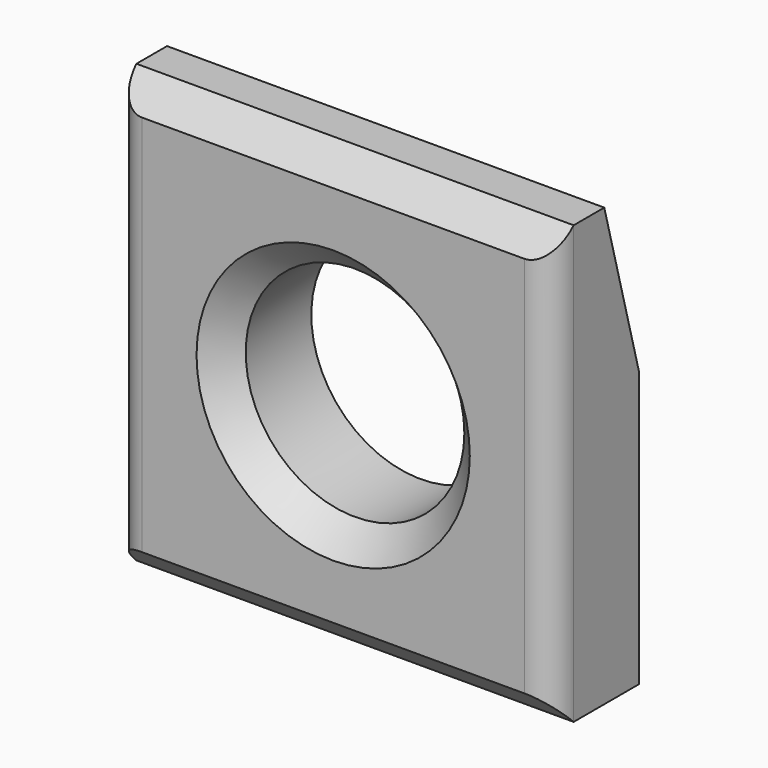
from build123d import *

# Parameters (mm, degrees)
F0_W        = 50.8
F0_H        = 50.8
F1_DEPTH    = 12.7
F2_R        = 12.7
F3_DEPTH    = 25.4
F4_R        = 3.175
F5_T1_DEPTH = 60.7801869736
F6_T1_DEPTH = 149.2615438243


# Not quite as in the source:
# - a fillet or chamfer that OpenCascade refuses, or shapes differently, is made with other operations: its cross-section is extruded or revolved along the edge and cut away or added


with BuildPart() as f1:
    # F0 (on Front) → F1 (new body)
    with BuildSketch(Plane.XZ):
        with Locations((25.4, -25.4)):
            Rectangle(F0_W, F0_H)
    extrude(amount=F1_DEPTH)

    # F2 (on face) → F3 (cut)
    with BuildSketch(Plane.XZ.offset(12.7)):
        with Locations((25.4, -25.4)):
            Circle(F2_R)
    extrude(amount=-F3_DEPTH, mode=Mode.SUBTRACT)

    # F4
    f4_edges = [f1.edges().sort_by_distance(p)[0] for p in [
        (0, -12.7, -25.4),
        (50.8, -12.7, -25.4),
    ]]
    fillet(f4_edges, radius=F4_R)

    # F5: chamfer of 3.175 on 3 edges, made by hand

    # F5_s2 → F5_t1 (cut)
    with BuildSketch(Plane.YZ.offset(-4.9900934868)):
        Polygon((-9.525, 0), (-12.7, -3.175), (-12.7, 0), align=None)
        Polygon((-12.7, -47.625), (-9.525, -50.8), (-12.7, -50.8), align=None)
    extrude(amount=F5_T1_DEPTH, mode=Mode.SUBTRACT)

    # F5_s3 → F5_t4 (revolve, cut)
    with BuildSketch(Plane.XY.offset(-25.4)):
        Polygon((41.275, -12.7), (38.1, -9.525), (38.1, -12.7), align=None)
    revolve(axis=Axis((25.4, -12.7, -25.4), (0, -1, 0)), mode=Mode.SUBTRACT)

    # F6: chamfer of 5.08 x 18.9588181024 on 1 edges, made by hand

    # F6_s2 → F6_t1 (cut)
    with BuildSketch(Plane.YZ.offset(-49.2307719121)):
        Polygon((-5.08, 0), (0, -18.9588181024), (0, 0), align=None)
    extrude(amount=F6_T1_DEPTH, mode=Mode.SUBTRACT)


solid = f1.part
